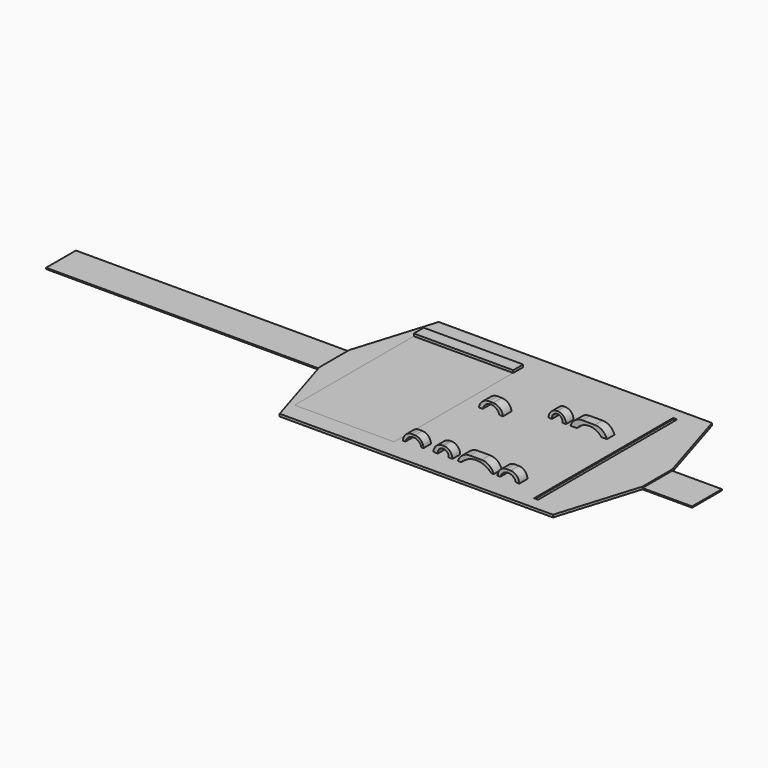
from build123d import *

# Parameters (mm, degrees)
F0_W         = 279.4
F0_H         = 38.1
F1_DEPTH     = 1.27
F3_DEPTH     = 2.54
F4_W         = 101.6
F4_H         = 165.1
F5_DEPTH     = 2.54
F6_W         = 101.6
F6_H         = 12.7
F7_DEPTH     = 2.54
F8_W         = 50.8
F8_H         = 38.1
F9_DEPTH     = 2.54
F10_W        = 50.8
F10_H        = 38.1
F11_DEPTH    = 1.27
F12_W        = 4.1427978277
F12_H        = 177.8
F13_DEPTH    = 1.27
F15_W        = 20.9306627512
F15_H        = 9.5325633883
F15_W_2      = 19.3549990654
F15_H_2      = 9.9495388567
F15_W_3      = 24.6197581291
F15_H_3      = 11.048823595
F15_W_4      = 36.6368442774
F15_H_4      = 10.3682503104
F15_W_5      = 17.9531574249
F15_H_5      = 9.6851810813
F15_W_6      = 37.1780246496
F15_H_6      = 9.7587406635
F15_W_7      = 21.9638049603
F15_H_7      = 10.8560696244
F16_DEPTH    = 8.89
F17_R        = 8.88999
F18_T1_DEPTH = 61.4503860708
F19_T1_DEPTH = 70.9433896004
F19_T3_DEPTH = 70.3338799535
F21_DEPTH    = 25.4
F23_DEPTH    = 25.4
F25_DEPTH    = 25.4
F26_W        = 21.9202637672
F26_H        = 0.403650105
F27_DEPTH    = 8.89
F29_DEPTH    = 25.4


# Not quite as in the source:
# - a fillet or chamfer that OpenCascade refuses, or shapes differently, is made with other operations: its cross-section is extruded or revolved along the edge and cut away or added
# - a fillet or chamfer is up to 0.001 mm smaller than in the source, because OpenCascade refuses the exact size


with BuildPart() as f1:
    # F0 (on Top) → F1 (new body)
    with BuildSketch(Plane.XY):
        with Locations((-165.1, 19.05)):
            Rectangle(F0_W, F0_H)
    extrude(amount=F1_DEPTH)

    # F2 (on Top) → F3 (join)
    with BuildSketch(Plane.XY):
        Polygon((0, -63.5), (0, 0), (0, 38.1), (0, 101.6), (0, 120.65), (-25.4, 38.1), (-25.4, 0), (0, -82.55), align=None)
        Polygon((101.6, -63.5), (0, -63.5), (0, -82.55), (279.4, -82.55), (279.4, 120.65), (0, 120.65), (0, 101.6), (101.6, 101.6), align=None)
        Polygon((279.4, 120.65), (279.4, -82.55), (304.8, 0), (304.8, 38.1), align=None)
    extrude(amount=F3_DEPTH)

    # F8 (on face) → F9 (join)
    with BuildSketch(Plane.XY.offset(2.54)):
        with Locations((330.2, 19.05)):
            Rectangle(F8_W, F8_H)
    extrude(amount=-F9_DEPTH)

    # F10 (on face) → F11 (cut)
    with BuildSketch(Plane.XY.offset(2.54)):
        with Locations((330.2, 19.05)):
            Rectangle(F10_W, F10_H)
    extrude(amount=-F11_DEPTH, mode=Mode.SUBTRACT)

    # F12 (on face) → F13 (cut)
    with BuildSketch(Plane.XY.offset(2.54)):
        with Locations((251.9286010861, 19.05)):
            Rectangle(F12_W, F12_H)
    extrude(amount=-F13_DEPTH, mode=Mode.SUBTRACT)

    # F15 (on face) → F16 (join)
    with BuildSketch(Plane.XY.offset(2.54)):
        with Locations((116.4400056005, -52.6323951781)):
            Rectangle(F15_W, F15_H)
        with Locations((146.8468159437, -52.4239074439)):
            Rectangle(F15_W_2, F15_H_2)
        with Locations((129.7524869442, 30.801191926)):
            Rectangle(F15_W_3, F15_H_3)
        with Locations((180.3798153996, -52.214551717)):
            Rectangle(F15_W_4, F15_H_4)
        with Locations((180.7809472084, 51.05381459)):
            Rectangle(F15_W_5, F15_H_5)
        with Locations((212.849445641, 51.0905943811)):
            Rectangle(F15_W_6, F15_H_6)
        with Locations((213.8880491257, -52.458461374)):
            Rectangle(F15_W_7, F15_H_7)
    extrude(amount=F16_DEPTH)

    # F17 (radius 8.89 in the source; OpenCascade refuses exactly that, so slightly less here)
    f17_edges = [f1.edges().sort_by_distance(p)[0] for p in [
        (105.974674, -52.632395, 11.43),
        (126.905337, -52.632395, 11.43),
        (137.169316, -52.423907, 11.43),
        (156.524315, -52.423907, 11.43),
        (202.906147, -52.458461, 11.43),
        (224.869952, -52.458461, 11.43),
        (189.757526, 51.053815, 11.43),
        (171.804368, 51.053815, 11.43),
    ]]
    fillet(f17_edges, radius=F17_R)

    # F18: fillet of radius 10.16 on 2 edges, made by hand

    # F18_s2 → F18_t1 (cut)
    with BuildSketch(Plane.XZ.offset(-61.5263849614)):
        with BuildLine():
            ThreePointArc((117.4426078796, 2.54), (120.8027120447, 8.89), (127.5229203748, 11.43))
            Line((127.5229203748, 11.43), (117.4426078796, 11.43))
            Line((117.4426078796, 11.43), (117.4426078796, 2.54))
        make_face()
        with BuildLine():
            ThreePointArc((142.0623660088, 2.54), (138.7022618437, 8.89), (131.9820535136, 11.43))
            Line((131.9820535136, 11.43), (142.0623660088, 11.43))
            Line((142.0623660088, 11.43), (142.0623660088, 2.54))
        make_face()
    extrude(amount=F18_T1_DEPTH, mode=Mode.SUBTRACT)

    # F19: fillet of radius 12.7 on 4 edges, made by hand

    # F19_s2 → F19_t1 (cut)
    with BuildSketch(Plane.XZ.offset(16.7428569168)):
        with BuildLine():
            ThreePointArc((162.061393261, 2.54), (166.6629997944, 8.9690673403), (174.176421119, 11.43))
            Line((174.176421119, 11.43), (162.061393261, 11.43))
            Line((162.061393261, 11.43), (162.061393261, 2.54))
        make_face()
        with BuildLine():
            ThreePointArc((198.6982375383, 2.54), (194.0966310049, 8.9690673403), (186.5832096803, 11.43))
            Line((186.5832096803, 11.43), (198.6982375383, 11.43))
            Line((198.6982375383, 11.43), (198.6982375383, 2.54))
        make_face()
    extrude(amount=F19_T1_DEPTH, mode=Mode.SUBTRACT)

    # F19_s4 → F19_t3 (cut)
    with BuildSketch(Plane.XZ.offset(-86.2575343578)):
        with BuildLine():
            ThreePointArc((194.2604333162, 2.54), (198.8620398497, 8.9690673403), (206.3754611742, 11.43))
            Line((206.3754611742, 11.43), (194.2604333162, 11.43))
            Line((194.2604333162, 11.43), (194.2604333162, 2.54))
        make_face()
        with BuildLine():
            ThreePointArc((231.4384579659, 2.54), (226.8368514324, 8.9690673403), (219.3234301079, 11.43))
            Line((219.3234301079, 11.43), (231.4384579659, 11.43))
            Line((231.4384579659, 11.43), (231.4384579659, 2.54))
        make_face()
    extrude(amount=F19_T3_DEPTH, mode=Mode.SUBTRACT)

    # F20 (on face) → F21 (cut)
    with BuildSketch(Plane.XZ.offset(-25.2767801285)):
        with BuildLine():
            Line((121.3961169124, 2.54), (138.3046656847, 2.54))
            ThreePointArc((138.3046656847, 2.54), (129.8503912985, 9.3004488884), (121.3961169124, 2.54))
        make_face()
    extrude(amount=-F21_DEPTH, mode=Mode.SUBTRACT)

    # F22 (on face) → F23 (cut)
    with BuildSketch(Plane.XZ.offset(-46.2112240493)):
        with BuildLine():
            Line((175.4323393106, 2.54), (186.2645745277, 2.54))
            ThreePointArc((186.2645745277, 2.54), (180.8484569192, 8.7688172062), (175.4323393106, 2.54))
        make_face()
        with BuildLine():
            Line((200.9464204311, 2.54), (226.0337024927, 2.54))
            ThreePointArc((226.0337024927, 2.54), (213.4900614619, 8.6103858863), (200.9464204311, 2.54))
        make_face()
    extrude(amount=-F23_DEPTH, mode=Mode.SUBTRACT)

    # F24 (on face) → F25 (cut)
    with BuildSketch(Plane.XZ.offset(57.3986768723)):
        with BuildLine():
            Line((108.5784949401, 2.54), (124.7587874532, 2.54))
            ThreePointArc((124.7587874532, 2.54), (116.6686411966, 9.025935128), (108.5784949401, 2.54))
        make_face()
        with BuildLine():
            Line((141.620144248, 2.54), (152.6894122362, 2.54))
            ThreePointArc((152.6894122362, 2.54), (147.1547782421, 8.6968366243), (141.620144248, 2.54))
        make_face()
        with BuildLine():
            Line((165.6893789768, 2.54), (196.2613910437, 2.54))
            ThreePointArc((196.2613910437, 2.54), (180.9753850102, 9.3243519976), (165.6893789768, 2.54))
        make_face()
        with BuildLine():
            Line((206.5167725086, 2.54), (221.5484082699, 2.54))
            ThreePointArc((221.5484082699, 2.54), (214.0325903893, 8.531034918), (206.5167725086, 2.54))
        make_face()
    extrude(amount=-F25_DEPTH, mode=Mode.SUBTRACT)

    # F26 (on face) → F27 (cut)
    with BuildSketch(Plane.XY.offset(11.43)):
        with Locations((214.1792923212, -57.6846711338)):
            Rectangle(F26_W, F26_H)
    extrude(amount=-F27_DEPTH, mode=Mode.SUBTRACT)

    # F28 (on face) → F29 (cut)
    with BuildSketch(Plane.XZ.offset(57.4828460813)):
        with BuildLine():
            Line((205.711632967, 2.54), (221.426859498, 2.54))
            ThreePointArc((221.426859498, 2.54), (213.5692462325, 8.6267545228), (205.711632967, 2.54))
        make_face()
    extrude(amount=-F29_DEPTH, mode=Mode.SUBTRACT)


with BuildPart() as f5:
    # F4 (on face) → F5 (new body)
    with BuildSketch(Plane.XY.offset(2.54)):
        with Locations((50.8, 19.05)):
            Rectangle(F4_W, F4_H)
    extrude(amount=-F5_DEPTH)

    # F6 (on face) → F7 (join)
    with BuildSketch(Plane.XY.offset(2.54)):
        with Locations((50.8, 95.25)):
            Rectangle(F6_W, F6_H)
    extrude(amount=F7_DEPTH)


solid = Compound([f1.part, f5.part])
